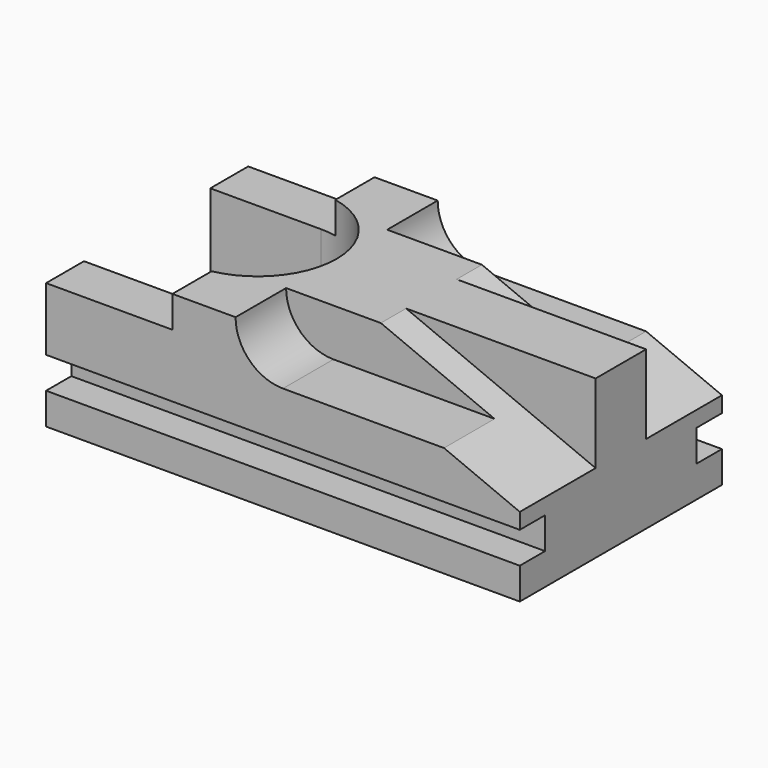
from build123d import *

# Parameters (mm, degrees)
F1_DEPTH = 50
F2_W     = 40
F2_H     = 10
F3_DEPTH = 30
F2_W_2   = 150
F4_DEPTH = 10
F5_DEPTH = 20


# Not quite as in the source:
# - a pattern or mirror of a feature is missing from the dataset's text; its kind, count and spacing are read off the source's solid


with BuildPart() as f1:
    # F0 (on Top) → F1 (new body)
    with BuildSketch(Plane.XY):
        with BuildLine():
            Line((-35, -25), (-35, -40))
            Line((-35, -40), (115, -40))
            Line((115, -40), (115, 40))
            Line((115, 40), (-35, 40))
            Line((-35, 40), (-35, 25))
            Line((-35, 25), (0, 25))
            ThreePointArc((0, 25), (25, 0), (0, -25))
            Line((0, -25), (-35, -25))
        make_face()
    extrude(amount=F1_DEPTH)

    # F2 (on face) → F3 (cut)
    with BuildSketch(Plane.XZ.offset(40)):
        with Locations((-15, 45)):
            Rectangle(F2_W, F2_H)
        Polygon((115, 50), (55, 50), (91, 35), (115, 25), align=None)
    f3 = extrude(amount=-F3_DEPTH, mode=Mode.SUBTRACT)

    # F3_copies: F3 across plane
    add(f3.mirror(Plane.ZX), mode=Mode.SUBTRACT)

    # F2 (on face) → F4 (cut)
    with BuildSketch(Plane.XZ.offset(40)):
        with Locations((40, 15)):
            Rectangle(F2_W_2, F2_H)
    f4 = extrude(amount=-F4_DEPTH, mode=Mode.SUBTRACT)

    # F4_copies: F4 across plane
    add(f4.mirror(Plane.ZX), mode=Mode.SUBTRACT)

    # F2 (on face) → F5 (cut)
    with BuildSketch(Plane.XZ.offset(40)):
        with BuildLine():
            Line((55, 50), (25, 50))
            ThreePointArc((25, 50), (29.3933982822, 39.3933982822), (40, 35))
            Line((40, 35), (91, 35))
            Line((91, 35), (55, 50))
        make_face()
    f5 = extrude(amount=-F5_DEPTH, mode=Mode.SUBTRACT)

    # F5_copies: F5 across plane
    add(f5.mirror(Plane.ZX), mode=Mode.SUBTRACT)


solid = f1.part
